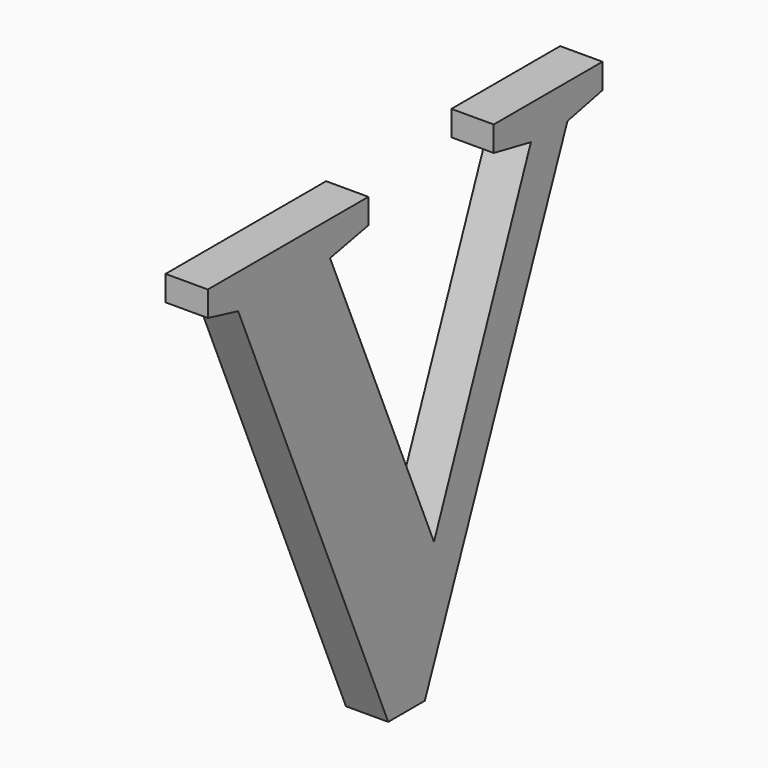
from build123d import *

# Parameters (mm, degrees)
F0_TEXT_SIZE = 635
F1_DEPTH     = 38.1


# Not quite as in the source:
# - Text() gives the source's letters only with a copy of the font that has no kerning and outlines rounded to 1/6400 em; it was checked with that copy


with BuildPart() as f1:
    # F0 (on Right) → F1 (new body)
    with BuildSketch(Plane.YZ):
        with Locations((-491.1328125, 0)):
            Text('V', F0_TEXT_SIZE, font='Tinos', font_style=FontStyle.BOLD, text_align=(TextAlign.LEFT, TextAlign.BOTTOM))
    extrude(amount=F1_DEPTH)


solid = f1.part
